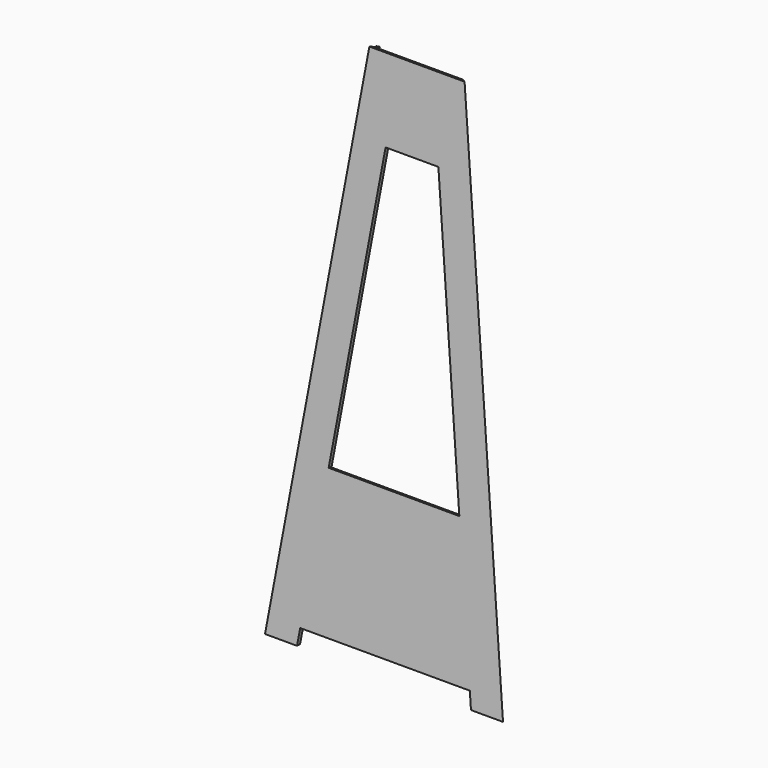
from build123d import *

# Parameters (mm, degrees)
F7_R      = 960.2431856589
F8_DEPTH  = 635.5163904251
F12_R     = 870.2287794889
F13_DEPTH = 25
F14_R     = 892.9375722879
F15_DEPTH = 25
F19_REACH = 935.9843056137
F20_DEPTH = 216.5073510461
F23_DEPTH = 25


with BuildPart() as f5:
    # F3 (on Top) → F5 section 0
    with BuildSketch(Plane.XY):
        Polygon((-375, -216.5063509461), (375, -216.5063509461), (0, 433.0127018922), align=None)
    # F4 (on line) → F5 section 1
    with BuildSketch(Plane.XY.offset(1650)):
        Polygon((-150, -86.6025403784), (150, -86.6025403784), (0, 173.2050807569), align=None)
    loft()

    # F7 (on face) → F8 (cut, through all)
    with BuildSketch(Plane(origin=(0, -203.2096543416, 15.9986111776), x_dir=(1, 0, 0), z_dir=(0, -0.9969151597, 0.078486714))):
        with Locations((0, 812.9688501358)):
            Circle(F7_R)
    extrude(amount=-F8_DEPTH, mode=Mode.SUBTRACT)

    # F12 (on face) → F13 (cut)
    with BuildSketch(Plane(origin=(0, 0, 0), x_dir=(0.8660254038, -0.5, 0), z_dir=(-0.5, -0.8660254038, 0))):
        with Locations((304.0688931942, 817.2121047974)):
            Circle(F12_R)
    extrude(amount=-F13_DEPTH, mode=Mode.SUBTRACT)

    # F14 (on face) → F15 (cut)
    with BuildSketch(Plane(origin=(0, 0, 0), x_dir=(-0.8660254038, -0.5, 0), z_dir=(-0.5, 0.8660254038, 0))):
        with Locations((291.6465699673, 811.1194968224)):
            Circle(F14_R)
    extrude(amount=F15_DEPTH, mode=Mode.SUBTRACT)

    f19_end = Plane(origin=(0, -155.5781982198, 697.4454188962), x_dir=(0, 0.078486714, 0.9969151597), z_dir=(0, 0.9969151597, -0.078486714))
    # F17 (on Front) → F19 (cut, up to a plane its end follows)
    with BuildSketch(Plane.XZ):
        Polygon((-181.3636363636, 1420), (181.3636363636, 1420), (179.7272727273, 1432), (-179.7272727273, 1432), align=None)
        Polygon((151.6363636364, 1638), (150, 1650), (-150, 1650), (-151.6363636364, 1638), align=None)
        Polygon((308.4545454545, 488), (306.8181818182, 500), (-306.8181818182, 500), (-308.4545454545, 488), align=None)
        Polygon((-365.4545454545, 70), (365.4545454545, 70), (363.8181818182, 82), (-363.8181818182, 82), align=None)
    f19_long = extrude(amount=F19_REACH, mode=Mode.PRIVATE)
    add(split(f19_long, bisect_by=f19_end, keep=Keep.TOP, mode=Mode.PRIVATE), mode=Mode.SUBTRACT)

    # F16 (on Front) → F20 (cut, through all)
    with BuildSketch(Plane.XZ):
        Polygon((-267.2563485856, 50), (-274.0745304038, 0), (274.0745304038, 0), (267.2563485856, 50), align=None)
        Polygon((-205.8927122219, 500), (205.8927122219, 500), (83.1654394947, 1400), (-83.1654394947, 1400), align=None)
    extrude(amount=F20_DEPTH, mode=Mode.SUBTRACT)

    # F22 (on face) → F23 (join)
    with BuildSketch(Plane(origin=(0, 0, 0), x_dir=(-0.8660254038, -0.5, 0), z_dir=(-0.5, 0.8660254038, 0))):
        Polygon((160.2172859615, 1639.4481457139), (151.0203254662, 1638), (153.2218541075, 1624.0184153092), (162.4188146029, 1625.4665610231), align=None)
    extrude(amount=F23_DEPTH)


solid = f5.part
